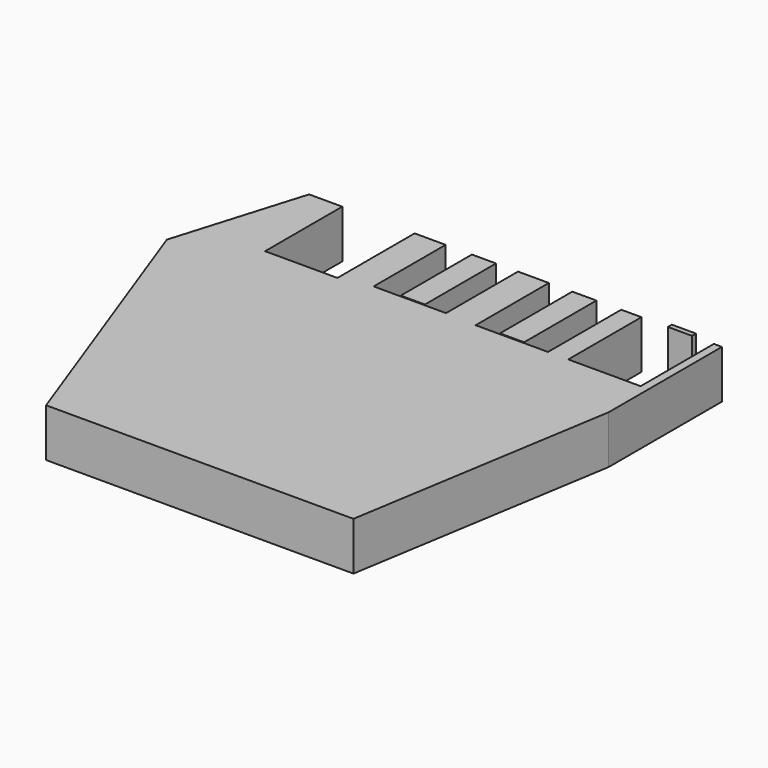
from build123d import *

# Parameters (mm, degrees)
F1_DEPTH = 10
F0_W     = 5
F0_H     = 1.0268185272
F0_H_2   = 18.4267202251
F0_H_3   = 18.7282770615


with BuildPart() as f1:
    # F0 (on Top) → F1 (new body)
    with BuildSketch(Plane.XY):
        Polygon((18.2068565833, -0.6069772576), (11.3289707911, -0.6069772576), (3.2589579517, -27.3683114747), (24.2683672618, -84.9190409688), (87.9804774548, -84.9190409688), (96.9007899468, -29.943118357), (96.9007899468, -0.6069772576), (95.2245366573, -0.6069772576), (95.2245366573, -19.5801587304), (90.7042622566, -19.5801587304), (85.7042622566, -19.5801587304), (80.2245366573, -19.5801587304), (80.2245366573, -0.6069772576), (76.032448262, -0.6069772576), (76.032448262, -19.5801581338), (61.032448262, -19.5801581338), (61.032448262, -0.6069772576), (54.6379645169, -0.6069772576), (54.6379645169, -19.2655338085), (39.6379645169, -19.2655338085), (39.6379645169, -0.6069772576), (33.2068565833, -0.6069772576), (33.2068565833, -20.6069772576), (27.8533260524, -20.6069772576), (22.8533260524, -20.6069772576), (18.2068565833, -20.6069772576), align=None)
    extrude(amount=F1_DEPTH)


with BuildPart() as f1b:
    # F0 (on Top) → F1, piece 2 (new body)
    with BuildSketch(Plane.XY):
        with Locations((88.2042622566, -0.093567994)):
            Rectangle(F0_W, F0_H)
    extrude(amount=F1_DEPTH)


with BuildPart() as f1c:
    # F0 (on Top) → F1, piece 3 (new body)
    with BuildSketch(Plane.XY):
        with Locations((47.5812256336, -9.8203373701)):
            Rectangle(F0_W, F0_H_2)
    extrude(amount=F1_DEPTH)


with BuildPart() as f1d:
    # F0 (on Top) → F1, piece 4 (new body)
    with BuildSketch(Plane.XY):
        with Locations((68.3888345957, -9.9711157883)):
            Rectangle(F0_W, F0_H_3)
    extrude(amount=F1_DEPTH)


solid = Compound([f1.part, f1b.part, f1c.part, f1d.part])
